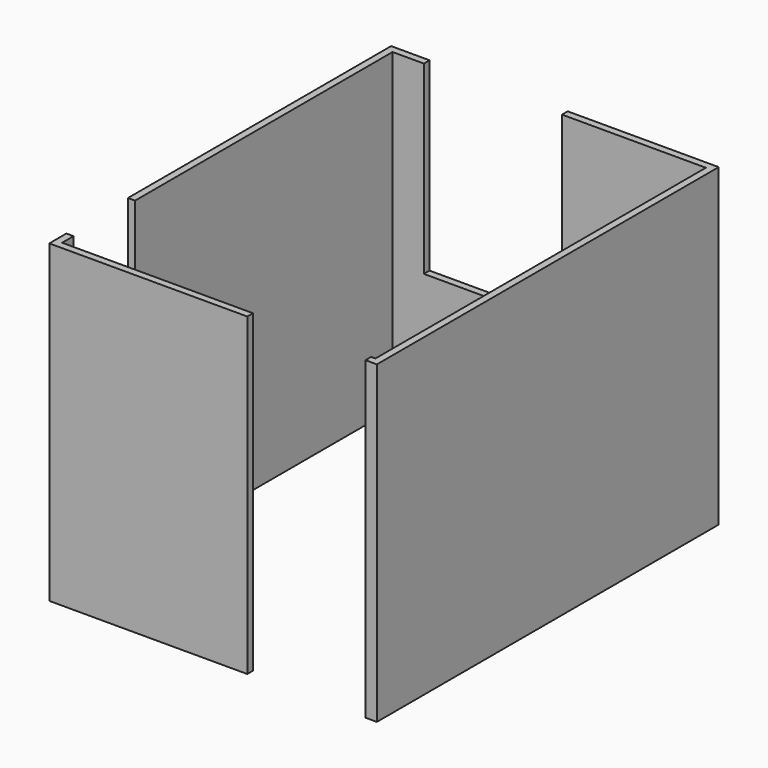
from build123d import *

# Parameters (mm, degrees)
F1_DEPTH = 890
F3_DEPTH = 20
F5_DEPTH = 1300


with BuildPart() as f1:
    # F0 (on Top) → F1 (new body)
    with BuildSketch(Plane.XY):
        Polygon((1100, 1450), (1100, -1450), (1070, -1450), (1070, -1500), (1150, -1500), (1150, 1500), (-1150, 1500), (-1150, -1500), (240, -1500), (240, -1450), (-1100, -1450), (-1100, 1450), align=None)
    extrude(amount=F1_DEPTH)

    # F2 (on face) → F3 (join)
    with BuildSketch(Plane.XY.offset(890)):
        Polygon((-1100, -1350), (-1150, -1350), (-1150, -1500), (240, -1500), (240, -1450), (-1100, -1450), align=None)
        Polygon((-1150, 1500), (-1150, -810), (-1100, -810), (-1100, 1450), (1100, 1450), (1100, -1450), (1070, -1450), (1070, -1500), (1150, -1500), (1150, 1500), align=None)
    extrude(amount=F3_DEPTH)

    # F3_face (on face) + F4 (on face) → F5 (join)
    with BuildSketch(Plane(origin=(107.2679045093, 530.198938992, 910), x_dir=(1, 0, 0), z_dir=(0, 0, 1))):
        Polygon((-1207.2679045093, -1880.198938992), (-1257.2679045093, -1880.198938992), (-1257.2679045093, -2030.198938992), (132.7320954907, -2030.198938992), (132.7320954907, -1980.198938992), (-1207.2679045093, -1980.198938992), align=None)
    with BuildSketch(Plane.XY.offset(910)):
        Polygon((-880, 1450), (-880, 1500), (-1150, 1500), (-1150, -810), (-1100, -810), (-1100, 1450), align=None)
        Polygon((1150, 1500), (90, 1500), (90, 1450), (1100, 1450), (1100, -1450), (1070, -1450), (1070, -1500), (1150, -1500), align=None)
    extrude(amount=F5_DEPTH)


solid = f1.part
